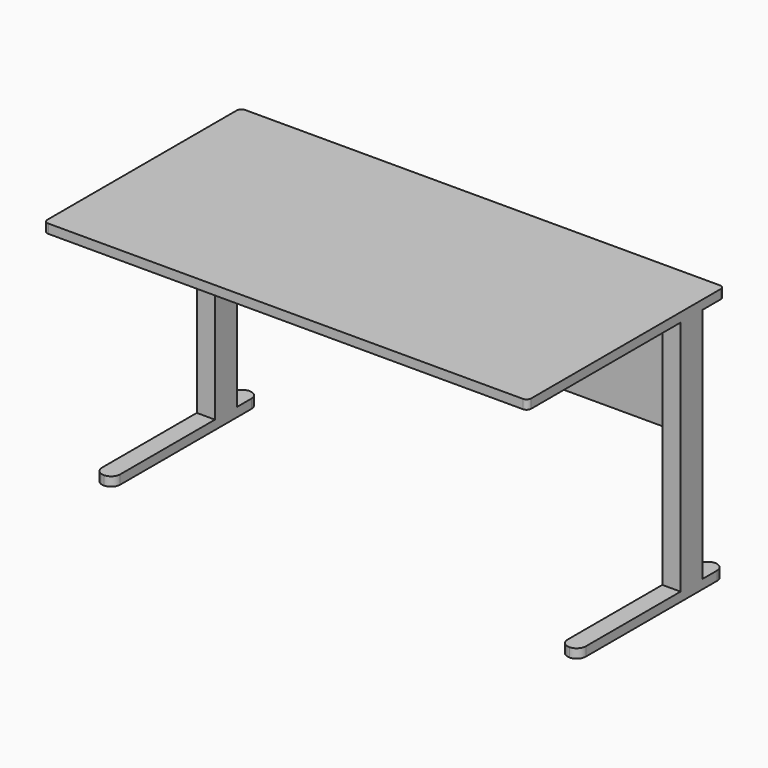
from build123d import *

# Parameters (mm, degrees)
F0_W     = 1348.74
F0_H     = 685.8
F1_DEPTH = 25.4
F2_W     = 50.8
F2_H     = 76.2
F3_DEPTH = 711.2
F4_W     = 508
F4_H     = 25.4
F4_W_2   = 76.2
F5_DEPTH = 50.8
F6_W     = 355.6
F6_H     = 25.4
F6_W_2   = 76.2
F7_DEPTH = 50.8
F8_W     = 1348.74
F8_H     = 25.4
F9_DEPTH = 304.8
F10_R    = 12.7
F11_R    = 25.39999


# Not quite as in the source:
# - a fillet or chamfer is up to 0.001 mm smaller than in the source, because OpenCascade refuses the exact size


with BuildPart() as f1:
    # F0 (on Top) → F1 (new body)
    with BuildSketch(Plane.XY):
        Rectangle(F0_W, F0_H)
    extrude(amount=F1_DEPTH)

    # F2 (on face) → F3 (join)
    with BuildSketch(Plane.XY.offset(25.4)):
        with Locations((-648.97, 228.6)):
            Rectangle(F2_W, F2_H)
        with Locations((648.97, 228.6)):
            Rectangle(F2_W, F2_H)
    extrude(amount=-F3_DEPTH)

    # F4 (on face) → F5 (join)
    with BuildSketch(Plane(origin=(-674.37, 0, 0), x_dir=(0, -1, 0), z_dir=(-1, 0, 0))):
        with Locations((-88.9, -673.1)):
            Rectangle(F4_W, F4_H)
        with Locations((-304.8, -673.1)):
            Rectangle(F4_W_2, F4_H)
    extrude(amount=-F5_DEPTH)

    # F6 (on face) → F7 (join)
    with BuildSketch(Plane.YZ.offset(674.37)):
        with Locations((12.7, -673.1)):
            Rectangle(F6_W, F6_H)
        with Locations((228.6, -673.1)):
            Rectangle(F6_W_2, F6_H)
        with Locations((304.8, -673.1)):
            Rectangle(F6_W_2, F6_H)
    extrude(amount=-F7_DEPTH)

    # F8 (on face) → F9 (join)
    with BuildSketch(Plane(origin=(0, 0, 0), x_dir=(1, 0, 0), z_dir=(0, 0, -1))):
        with Locations((0, -254)):
            Rectangle(F8_W, F8_H)
    extrude(amount=F9_DEPTH)

    # F10
    f10_edges = [f1.edges().sort_by_distance(p)[0] for p in [
        (674.37, -342.9, 12.7),
        (-674.37, -342.9, 12.7),
        (-674.37, 342.9, 12.7),
        (674.37, 342.9, 12.7),
    ]]
    fillet(f10_edges, radius=F10_R)

    # F11 (radius 25.4 in the source; OpenCascade refuses exactly that, so slightly less here)
    f11_edges = [f1.edges().sort_by_distance(p)[0] for p in [
        (-623.57, -165.1, -673.1),
        (-674.37, -165.1, -673.1),
        (674.37, -165.1, -673.1),
        (623.57, -165.1, -673.1),
        (674.37, 342.9, -673.1),
        (623.57, 342.9, -673.1),
        (-674.37, 342.9, -673.1),
        (-623.57, 342.9, -673.1),
    ]]
    fillet(f11_edges, radius=F11_R)


solid = f1.part
